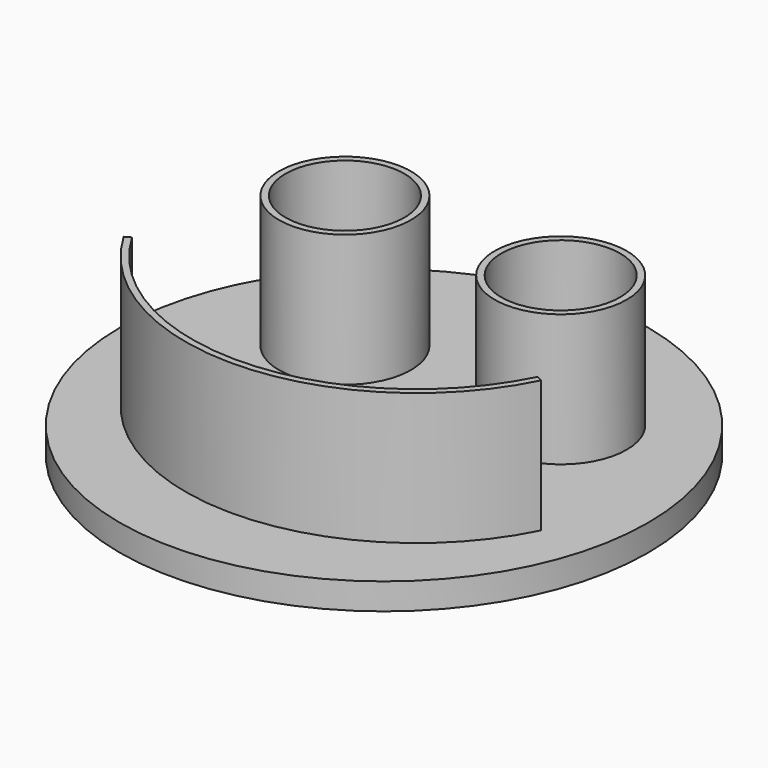
from build123d import *

# Parameters (mm, degrees)
F0_R     = 40
F1_DEPTH = 4
F3_DEPTH = 20
F4_R     = 10
F4_R_2   = 9
F5_DEPTH = 20


with BuildPart() as f1:
    # F0 (on Top) → F1 (new body)
    with BuildSketch(Plane.XY):
        Circle(F0_R)
    extrude(amount=F1_DEPTH)

    # F2 (on face) → F3 (join)
    with BuildSketch(Plane.XY.offset(4)):
        with BuildLine():
            Line((-29.3314530519, -11.0355725728), (-30.1941428334, -11.5413060412))
            ThreePointArc((-30.1941428334, -11.5413060412), (1.2017746888, -28.8199962275), (31.3377837192, -9.4272725577))
            Line((31.3377837192, -9.4272725577), (30.4424184562, -8.981940046))
            ThreePointArc((30.4424184562, -8.981940046), (1.1674382553, -27.8205858967), (-29.3314530519, -11.0355725728))
        make_face()
    extrude(amount=F3_DEPTH)



with BuildPart() as f5:
    # F4 (on face) → F5 (new body)
    with BuildSketch(Plane.XY.offset(4)):
        with Locations((16.3378193974, 13.0289122462)):
            Circle(F4_R)
        with Locations((16.3378193974, 13.0289122462)):
            Circle(F4_R_2, mode=Mode.SUBTRACT)
    extrude(amount=F5_DEPTH)


with BuildPart() as f1_1:
    add(f1.part)

    add(f5.part)  # F6 merges F5
    # F6: F5 across plane
    add(f5.part.mirror(Plane.YZ))


solid = f1_1.part
